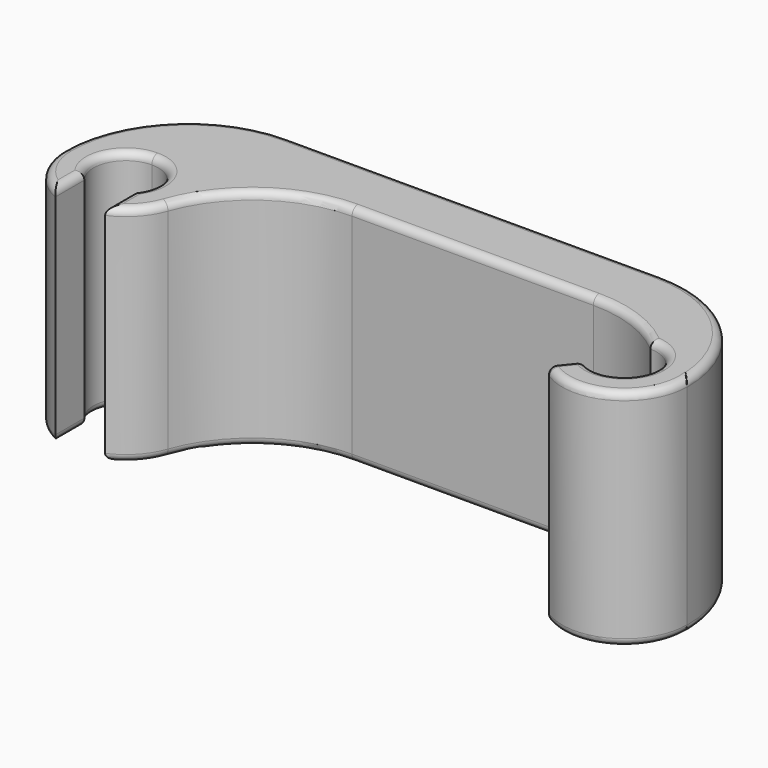
from build123d import *

# Parameters (mm, degrees)
F1_DEPTH    = 9
F2_T1_DEPTH = 9
F2_T3_DEPTH = 9
F2_T5_DEPTH = 34
F2_T7_DEPTH = 34
F3_R        = 0.3


# Not quite as in the source:
# - a fillet or chamfer that OpenCascade refuses, or shapes differently, is made with other operations: its cross-section is extruded or revolved along the edge and cut away or added


with BuildPart() as f1:
    # F0 (on Top) → F1 (new body)
    with BuildSketch(Plane.XY):
        with BuildLine():
            Line((-2.5, 5), (-2.5, 0))
            ThreePointArc((-2.5, 0), (-2.0916500663, -1.3693063938), (-1, -2.2912878475))
            Line((-1, -2.2912878475), (-1, -0.8306623863))
            ThreePointArc((-1, -0.8306623863), (-1.1768307232, 0.5523309234), (0, 1.3))
            ThreePointArc((0, 1.3), (1.1768307232, 0.5523309234), (1, -0.8306623863))
            Line((1, -0.8306623863), (1, -2.2912878475))
            ThreePointArc((1, -2.2912878475), (2.0916500663, -1.3693063938), (2.5, 0))
            Line((2.5, 0), (2.5, 2.5))
            Line((2.5, 2.5), (20, 2.5))
            ThreePointArc((20, 2.5), (21.767766953, 1.767766953), (22.5, 0))
            Line((22.5, 0), (22.5134724528, 0))
            Line((22.5134724528, 0), (22.5134724528, 5))
            Line((22.5134724528, 5), (-2.5, 5))
        make_face()
        with BuildLine():
            ThreePointArc((18.4241019781, -1.9407589815), (21.074768567, -2.2571824311), (22.5, 0))
            Line((22.5, 0), (21.3, 0))
            ThreePointArc((21.3, 0), (20.5588796548, -1.1737348642), (19.1805330286, -1.0091946704))
            Line((19.1805330286, -1.0091946704), (18.4241019781, -1.9407589815))
        make_face()
        with BuildLine():
            Line((21.3, 0), (22.5, 0))
            ThreePointArc((22.5, 0), (21.767766953, 1.767766953), (20, 2.5))
            Line((20, 2.5), (20, 1.3))
            ThreePointArc((20, 1.3), (20.9192388155, 0.9192388155), (21.3, 0))
        make_face()
    extrude(amount=F1_DEPTH)

    # F2: fillet of radius 5 on 4 edges, made by hand

    # F2_s2 → F2_t1 (join)
    with BuildSketch(Plane.XY):
        with BuildLine():
            ThreePointArc((2.357022604, -0.8333333333), (4.1843164659, 1.5824829046), (7.0710678119, 2.5))
            Line((7.0710678119, 2.5), (7.0710678119, 3))
            Line((7.0710678119, 3), (2.5, 3))
            Line((2.5, 3), (2, 2.5))
            ThreePointArc((2, 2.5), (2, 0), (1.8856180832, -0.6666666667))
            Line((1.8856180832, -0.6666666667), (2.357022604, -0.8333333333))
        make_face()
    extrude(amount=F2_T1_DEPTH)

    # F2_s4 → F2_t3 (join)
    with BuildSketch(Plane.XY):
        with BuildLine():
            ThreePointArc((20, 1.3), (18.4824354457, 2.1904157598), (16.7503846381, 2.5))
            Line((16.7503846381, 2.5), (20, 2.5))
            Line((20, 2.5), (20, 1.3))
        make_face()
    extrude(amount=F2_T3_DEPTH)

    # F2_s6 → F2_t5 (cut)
    with BuildSketch(Plane.XY.offset(-12.5)):
        with BuildLine():
            ThreePointArc((-2.5, 0), (-1.0355339059, 3.5355339059), (2.5, 5))
            Line((2.5, 5), (-2.5, 5))
            Line((-2.5, 5), (-2.5, 0))
        make_face()
    extrude(amount=F2_T5_DEPTH, mode=Mode.SUBTRACT)

    # F2_s8 → F2_t7 (cut)
    with BuildSketch(Plane.XY.offset(-12.5)):
        with BuildLine():
            ThreePointArc((17.5134724528, 5), (21.0490063587, 3.5355339059), (22.5134724528, 0))
            Line((22.5134724528, 0), (22.5134724528, 5))
            Line((22.5134724528, 5), (17.5134724528, 5))
        make_face()
    extrude(amount=F2_T7_DEPTH, mode=Mode.SUBTRACT)

    # F3
    f3_edges = [f1.edges().sort_by_distance(p)[0] for p in [
        (22.506736, 0, 9),
        (21.074769, -2.257182, 9),
        (18.802318, -1.474977, 9),
        (21.225143, -0.434768, 9),
        (18.482435, 2.190416, 9),
        (11.910726, 2.5, 9),
        (4.184316, 1.582483, 9),
        (1.829975, -1.703289, 9),
        (1, -1.560975, 9),
        (0, 1.3, 9),
        (-1, -1.560975, 9),
        (-2.09165, -1.369306, 9),
        (-1.035534, 3.535534, 9),
        (10.006736, 5, 9),
        (21.049006, 3.535534, 9),
        (22.506736, 0, 0),
        (21.074769, -2.257182, 0),
        (18.802318, -1.474977, 0),
        (21.225143, -0.434768, 0),
        (18.482435, 2.190416, 0),
        (11.910726, 2.5, 0),
        (4.184316, 1.582483, 0),
        (1.829975, -1.703289, 0),
        (1, -1.560975, 0),
        (0, 1.3, 0),
        (-1, -1.560975, 0),
        (-2.09165, -1.369306, 0),
        (-1.035534, 3.535534, 0),
        (10.006736, 5, 0),
        (21.049006, 3.535534, 0),
        (19.180533, -1.009195, 4.5),
        (18.424102, -1.940759, 4.5),
    ]]
    fillet(f3_edges, radius=F3_R)


solid = f1.part
